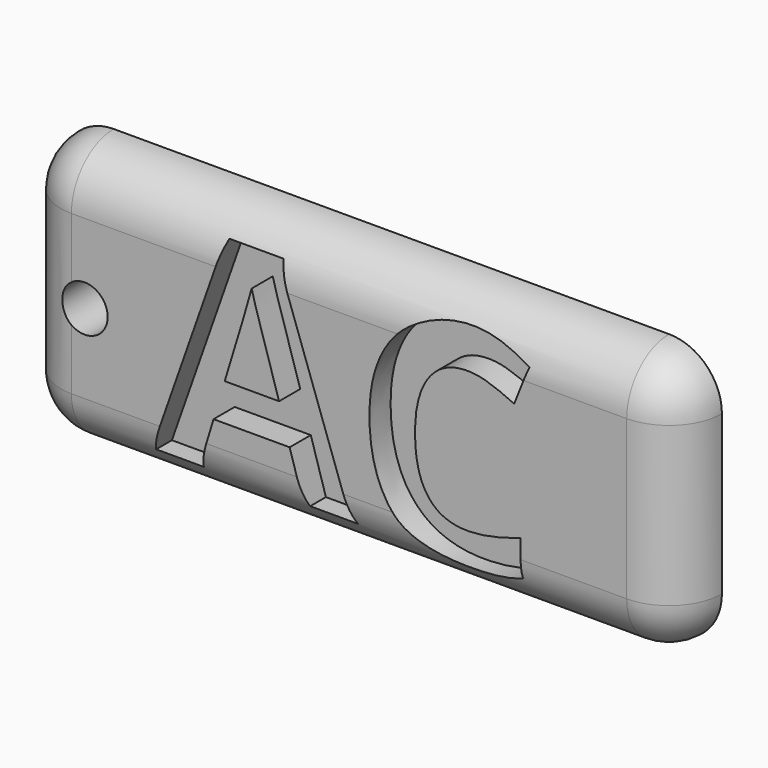
from build123d import *

# Parameters (mm, degrees)
F0_W         = 63.5
F0_H         = 25.4
F1_DEPTH     = 5.08
F2_R         = 5.08
F3_R         = 2.2117559802
F4_DEPTH     = 5.081
F5_TEXT_SIZE = 28.0792261631
F6_DEPTH     = 2.54
F7_T1_DEPTH  = 15.24
F7_T3_DEPTH  = 53.34
F7_T6_ANGLE  = 90
F7_T8_ANGLE  = 90
F7_T10_ANGLE = 90
F7_T12_ANGLE = 90


# Not quite as in the source:
# - a fillet or chamfer that OpenCascade refuses, or shapes differently, is made with other operations: its cross-section is extruded or revolved along the edge and cut away or added
# - Text() gives the source's letters only with a copy of the font that has no kerning and outlines rounded to 1/6400 em; it was checked with that copy


with BuildPart() as f1:
    # F0 (on Front) → F1 (new body)
    with BuildSketch(Plane.XZ):
        Rectangle(F0_W, F0_H)
    extrude(amount=F1_DEPTH)

    # F2
    f2_edges = [f1.edges().sort_by_distance(p)[0] for p in [
        (31.75, -2.54, 12.7),
        (31.75, -2.54, -12.7),
        (-31.75, -2.54, 12.7),
        (-31.75, -2.54, -12.7),
    ]]
    fillet(f2_edges, radius=F2_R)

    # F3 (on face) → F4 (cut, through all)
    with BuildSketch(Plane.XZ.offset(5.08)):
        with Locations((-25.4, 0)):
            Circle(F3_R)
    extrude(amount=-F4_DEPTH, mode=Mode.SUBTRACT)

    # F5 (on face) → F6 (cut)
    with BuildSketch(Plane.XZ.offset(5.08)):
        with Locations((-19.05, -10.1078428374)):
            Text('AC', F5_TEXT_SIZE, font='Open Sans', font_style=FontStyle.BOLD, text_align=(TextAlign.LEFT, TextAlign.BOTTOM))
    extrude(amount=-F6_DEPTH, mode=Mode.SUBTRACT)

    # F7: fillet of radius 5.08 on 1 edges, made by hand

    # F7_s2 → F7_t1 (cut)
    with BuildSketch(Plane.XY.offset(-7.62)):
        with BuildLine():
            ThreePointArc((26.67, -5.08), (30.2621024484, -3.5921024484), (31.75, 0))
            Line((31.75, 0), (31.75, -5.08))
            Line((31.75, -5.08), (26.67, -5.08))
        make_face()
        with BuildLine():
            ThreePointArc((-26.67, -5.08), (-30.2621024484, -3.5921024484), (-31.75, 0))
            Line((-31.75, 0), (-31.75, -5.08))
            Line((-31.75, -5.08), (-26.67, -5.08))
        make_face()
    extrude(amount=F7_T1_DEPTH, mode=Mode.SUBTRACT)

    # F7_s4 → F7_t3 (cut)
    with BuildSketch(Plane.YZ.offset(-26.67)):
        with BuildLine():
            ThreePointArc((0, 12.7), (-3.5921024484, 11.2121024484), (-5.08, 7.62))
            Line((-5.08, 7.62), (-5.08, 12.7))
            Line((-5.08, 12.7), (0, 12.7))
        make_face()
        with BuildLine():
            ThreePointArc((-5.08, -7.62), (-3.5921024484, -11.2121024484), (0, -12.7))
            Line((0, -12.7), (-5.08, -12.7))
            Line((-5.08, -12.7), (-5.08, -7.62))
        make_face()
    extrude(amount=F7_T3_DEPTH, mode=Mode.SUBTRACT)

    # F7_s5 → F7_t6 (revolve, cut)
    with BuildSketch(Plane.YZ.offset(26.67)):
        with BuildLine():
            ThreePointArc((-5.08, -7.62), (-3.5921024484, -11.2121024484), (0, -12.7))
            Line((0, -12.7), (-5.08, -12.7))
            Line((-5.08, -12.7), (-5.08, -7.62))
        make_face()
    revolve(axis=Axis((26.67, -5.08, -7.62), (0, -1, 0)), revolution_arc=F7_T6_ANGLE, mode=Mode.SUBTRACT)

    # F7_s7 → F7_t8 (revolve, cut)
    with BuildSketch(Plane.YZ.offset(26.67)):
        with BuildLine():
            ThreePointArc((0, 12.7), (-3.5921024484, 11.2121024484), (-5.08, 7.62))
            Line((-5.08, 7.62), (-5.08, 12.7))
            Line((-5.08, 12.7), (0, 12.7))
        make_face()
    revolve(axis=Axis((26.67, -5.08, 7.62), (0, 1, 0)), revolution_arc=F7_T8_ANGLE, mode=Mode.SUBTRACT)

    # F7_s9 → F7_t10 (revolve, cut)
    with BuildSketch(Plane.YZ.offset(-26.67)):
        with BuildLine():
            ThreePointArc((0, 12.7), (-3.5921024484, 11.2121024484), (-5.08, 7.62))
            Line((-5.08, 7.62), (-5.08, 12.7))
            Line((-5.08, 12.7), (0, 12.7))
        make_face()
    revolve(axis=Axis((-26.67, -5.08, 7.62), (0, -1, 0)), revolution_arc=F7_T10_ANGLE, mode=Mode.SUBTRACT)

    # F7_s11 → F7_t12 (revolve, cut)
    with BuildSketch(Plane.XY.offset(-7.62)):
        with BuildLine():
            ThreePointArc((-26.67, -5.08), (-30.2621024484, -3.5921024484), (-31.75, 0))
            Line((-31.75, 0), (-31.75, -5.08))
            Line((-31.75, -5.08), (-26.67, -5.08))
        make_face()
    revolve(axis=Axis((-26.67, -5.08, -7.62), (0, -1, 0)), revolution_arc=F7_T12_ANGLE, mode=Mode.SUBTRACT)


solid = f1.part
